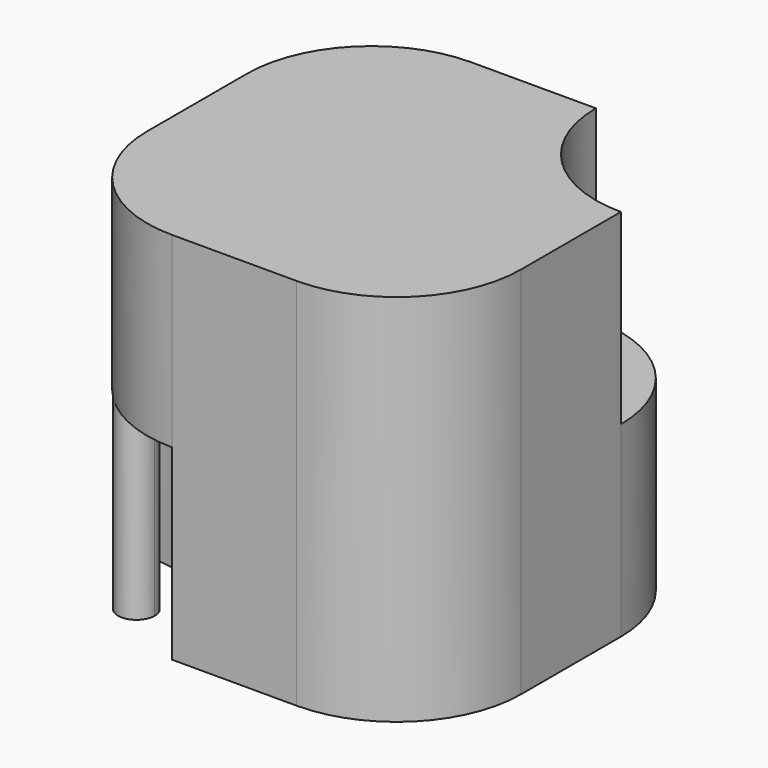
from build123d import *

# Parameters (mm, degrees)
F1_DEPTH = 304.8
F3_DEPTH = 304.8


# Not quite as in the source:
# - the program builds the solid bodies; features that only make, move or delete a surface that nothing else refers to are left out


with BuildPart() as f1:
    # F0 (on Top) → F1 (new body)
    with BuildSketch(Plane.XY):
        with BuildLine():
            Line((-101.6, -304.8), (101.6, -304.8))
            ThreePointArc((101.6, -304.8), (245.2840979371, -245.2840979371), (304.8, -101.6))
            Line((304.8, -101.6), (304.8, 101.6))
            ThreePointArc((304.8, 101.6), (161.1159020629, 161.1159020629), (101.6, 304.8))
            Line((101.6, 304.8), (-101.6, 304.8))
            ThreePointArc((-101.6, 304.8), (-245.2840979371, 245.2840979371), (-304.8, 101.6))
            Line((-304.8, 101.6), (-304.8, -101.6))
            ThreePointArc((-304.8, -101.6), (-161.1159020629, -161.1159020629), (-101.6, -304.8))
        make_face()
        with BuildLine():
            ThreePointArc((101.6, 304.8), (161.1159020629, 161.1159020629), (304.8, 101.6))
            ThreePointArc((304.8, 101.6), (245.2840979371, 245.2840979371), (101.6, 304.8))
        make_face()
    extrude(amount=F1_DEPTH)

    # F2 (on face) → F3 (join)
    with BuildSketch(Plane.XY.offset(304.8)):
        with BuildLine():
            Line((304.8, -101.6), (304.8, 101.6))
            ThreePointArc((304.8, 101.6), (161.1159020629, 161.1159020629), (101.6, 304.8))
            Line((101.6, 304.8), (-101.6, 304.8))
            ThreePointArc((-101.6, 304.8), (-245.2840979371, 245.2840979371), (-304.8, 101.6))
            Line((-304.8, 101.6), (-304.8, -101.6))
            ThreePointArc((-304.8, -101.6), (-245.2840979371, -245.2840979371), (-101.6, -304.8))
            Line((-101.6, -304.8), (101.6, -304.8))
            ThreePointArc((101.6, -304.8), (245.2840979371, -245.2840979371), (304.8, -101.6))
        make_face()
    extrude(amount=F3_DEPTH)


with BuildPart() as f1b:
    # F0 (on Top) → F1, piece 2 (new body)
    with BuildSketch(Plane.XY):
        with BuildLine():
            ThreePointArc((-194.4840979371, -224.2420489686), (-235.6299238094, -196.7492870811), (-245.2840979371, -245.2840979371))
            ThreePointArc((-245.2840979371, -245.2840979371), (-212.8541741277, -251.734810856), (-194.4840979371, -224.2420489686))
        make_face()
    extrude(amount=F1_DEPTH)


solid = Compound([f1.part, f1b.part])
